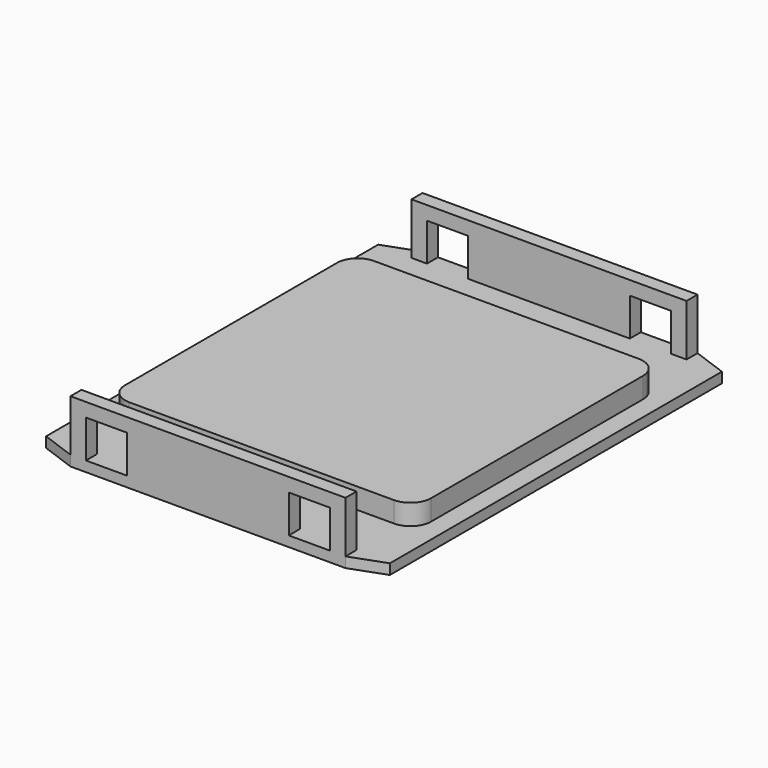
from build123d import *

# Parameters (mm, degrees)
F0_W         = 50
F0_H         = 60
F1_DEPTH     = 1.5
F2_W         = 20
F2_H         = 2
F3_DEPTH     = 9
F4_W         = 6
F4_H         = 5.5
F5_DEPTH     = 32
F6_W         = 44.5
F6_H         = 44.5
F7_DEPTH     = 4.5
F8_R         = 3
F9_T4_DEPTH  = 1.5
F9_T9_DEPTH  = 1.5
F9_T14_DEPTH = 1.5
F9_T19_DEPTH = 1.5


# Not quite as in the source:
# - a fillet or chamfer that OpenCascade refuses, or shapes differently, is made with other operations: its cross-section is extruded or revolved along the edge and cut away or added
# - a feature of the source that left no trace in its solid (it failed there, or was rolled back) is left out


with BuildPart() as f1:
    # F0 (on Top) → F1 (new body)
    with BuildSketch(Plane.XY):
        Rectangle(F0_W, F0_H)
    extrude(amount=F1_DEPTH)

    # F2 (on Top) → F3 (join)
    with BuildSketch(Plane.XY):
        with Locations((10, 31)):
            Rectangle(F2_W, F2_H)
        with Locations((-10, 31)):
            Rectangle(F2_W, F2_H)
        with Locations((-10, -31)):
            Rectangle(F2_W, F2_H)
        with Locations((10, -31)):
            Rectangle(F2_W, F2_H)
    extrude(amount=F3_DEPTH)

    # F4 (on Front) → F5 (cut, symmetric)
    with BuildSketch(Plane.XZ):
        with Locations((-14.75, 4.25)):
            Rectangle(F4_W, F4_H)
        with Locations((14.75, 4.25)):
            Rectangle(F4_W, F4_H)
    extrude(amount=F5_DEPTH, both=True, mode=Mode.SUBTRACT)

    # F6 (on Top) → F7 (join)
    with BuildSketch(Plane.XY):
        Rectangle(F6_W, F6_H)
    extrude(amount=F7_DEPTH)

    # F8
    f8_edges = [f1.edges().sort_by_distance(p)[0] for p in [
        (22.25, -22.25, 3),
        (-22.25, -22.25, 3),
        (-22.25, 22.25, 3),
        (22.25, 22.25, 3),
    ]]
    fillet(f8_edges, radius=F8_R)

    # F9: chamfer of 2 x 5.4949548389 on 4 edges, made by hand


with BuildPart() as f9_tool2:
    # F9_s3 → F9_t4 (new body)
    with BuildSketch(Plane.XY):
        Polygon((25.4949548389, 30), (20, 32), (20, 30), align=None)
    extrude(amount=F9_T4_DEPTH)

    split(bisect_by=Plane.YZ.offset(25), keep=Keep.BOTTOM)


with BuildPart() as f1_1:
    add(f1.part)

    # F9_t1: union F9_tool2
    add(f9_tool2.part)


with BuildPart() as f9_tool7:
    # F9_s8 → F9_t9 (new body)
    with BuildSketch(Plane.XY):
        Polygon((-25.4949548389, -30), (-20, -32), (-20, -30), align=None)
    extrude(amount=F9_T9_DEPTH)

    split(bisect_by=Plane.YZ.offset(-25), keep=Keep.TOP)


with BuildPart() as f1_2:
    add(f1_1.part)

    # F9_t6: union F9_tool7
    add(f9_tool7.part)


with BuildPart() as f9_tool12:
    # F9_s13 → F9_t14 (new body)
    with BuildSketch(Plane.XY):
        Polygon((-25.4949548389, 30), (-20, 32), (-20, 30), align=None)
    extrude(amount=F9_T14_DEPTH)

    split(bisect_by=Plane.YZ.offset(-25), keep=Keep.TOP)


with BuildPart() as f1_3:
    add(f1_2.part)

    # F9_t11: union F9_tool12
    add(f9_tool12.part)


with BuildPart() as f9_tool17:
    # F9_s18 → F9_t19 (new body)
    with BuildSketch(Plane.XY):
        Polygon((25.4949548389, -30), (20, -32), (20, -30), align=None)
    extrude(amount=F9_T19_DEPTH)

    split(bisect_by=Plane.YZ.offset(25), keep=Keep.BOTTOM)


with BuildPart() as f1_4:
    add(f1_3.part)

    # F9_t16: union F9_tool17
    add(f9_tool17.part)


solid = f1_4.part
